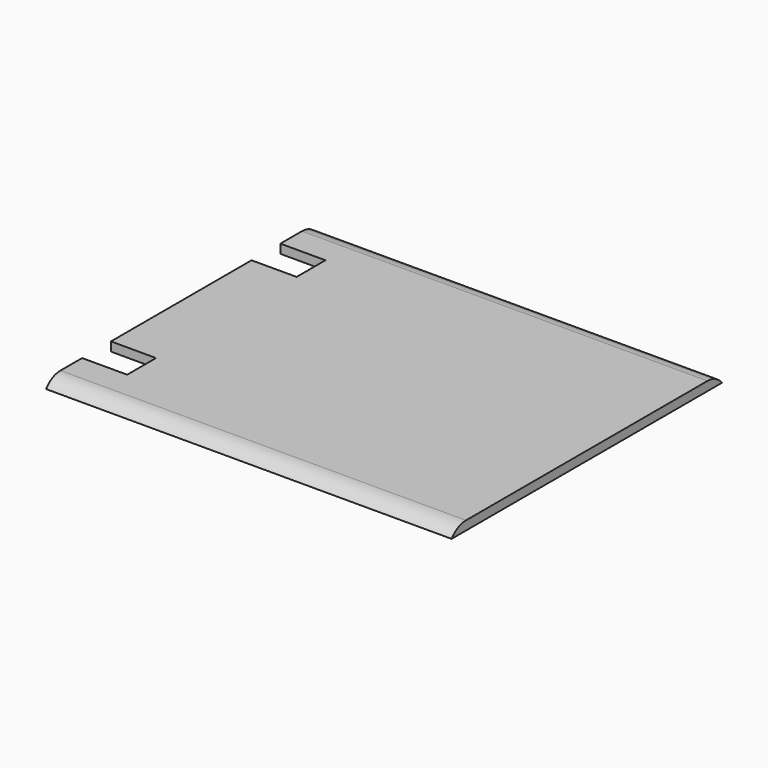
from build123d import *

# Parameters (mm, degrees)
F1_DEPTH    = 2
F2_T1_DEPTH = 110


# Not quite as in the source:
# - a fillet or chamfer that OpenCascade refuses, or shapes differently, is made with other operations: its cross-section is extruded or revolved along the edge and cut away or added


with BuildPart() as f1:
    # F0 (on Top) → F1 (new body)
    with BuildSketch(Plane.XY):
        Polygon((45, 27.5), (-35, 27.5), (-35, 19.5), (-45, 19.5), (-45, -19.5), (-35, -19.5), (-35, -27.5), (45, -27.5), align=None)
        Polygon((-45, 37.5), (-45, 27.5), (-35, 27.5), (45, 27.5), (45, 37.5), align=None)
        Polygon((45, -37.5), (45, -27.5), (-35, -27.5), (-45, -27.5), (-45, -37.5), align=None)
    extrude(amount=F1_DEPTH)

    # F2: fillet of radius 5 on 2 edges, made by hand

    # F2_s2 → F2_t1 (cut)
    with BuildSketch(Plane.YZ.offset(-55)):
        with BuildLine():
            ThreePointArc((37.5, 0), (35.7360679775, 1.472135955), (33.5, 2))
            Line((33.5, 2), (37.5, 2))
            Line((37.5, 2), (37.5, 0))
        make_face()
        with BuildLine():
            ThreePointArc((-37.5, 0), (-35.7360679775, 1.472135955), (-33.5, 2))
            Line((-33.5, 2), (-37.5, 2))
            Line((-37.5, 2), (-37.5, 0))
        make_face()
    extrude(amount=F2_T1_DEPTH, mode=Mode.SUBTRACT)


solid = f1.part
